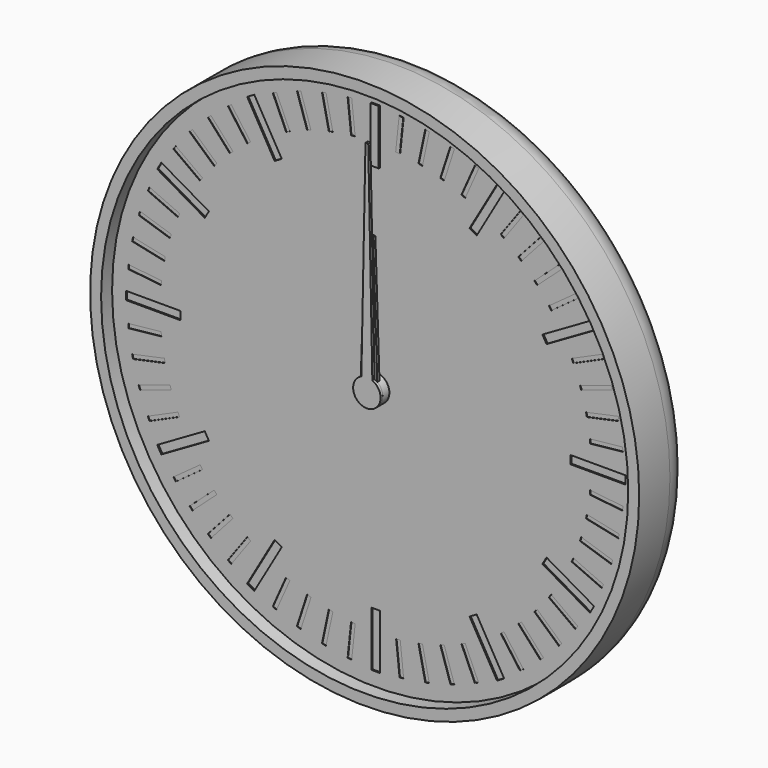
from build123d import *

# Parameters (mm, degrees)
F0_R      = 100
F1_DEPTH  = 24
F2_R      = 10
F3_T      = -4
F4_R      = 5
F4_R_2    = 3
F5_DEPTH  = 2
F6_DEPTH  = 19
F7_DEPTH  = 8
F9_DEPTH  = 4
F11_DEPTH = 4
F12_R     = 5
F12_R_2   = 3
F13_DEPTH = 2
F14_R     = 3
F15_DEPTH = 4
F17_DEPTH = 4
F18_R     = 3
F19_DEPTH = 2
F20_R     = 98
F20_R_2   = 5
F21_DEPTH = 1
F23_R     = 5
F23_R_2   = 3
F24_DEPTH = 2
F25_W     = 3
F25_H     = 20
F25_W_2   = 20
F25_H_2   = 3
F26_DEPTH = 0.5
F27_W     = 1.5
F27_H     = 12
F27_W_2   = 12
F27_H_2   = 1.5
F28_DEPTH = 0.2
F29_DEPTH = 1
F30_DEPTH = 0.4
F31_R     = 5
F31_R_2   = 3
F32_DEPTH = 5
F33_R     = 3
F34_DEPTH = 1
F36_DEPTH = 1


with BuildPart() as f1:
    # F0 (on Front) → F1 (new body)
    with BuildSketch(Plane.XZ):
        Circle(F0_R)
    extrude(amount=F1_DEPTH)

    # F2
    f2_edges = [f1.edges().sort_by_distance(p)[0] for p in [
        (-100, 0, 0),
    ]]
    fillet(f2_edges, radius=F2_R)

    # F3
    f3_openings = [f1.faces().sort_by_distance(p)[0] for p in [
        (0, -24, 0),
    ]]
    offset(amount=F3_T, openings=f3_openings)

    # F4 (on face) → F5 (join)
    with BuildSketch(Plane.XZ.offset(4)):
        Circle(F4_R)
        Circle(F4_R_2, mode=Mode.SUBTRACT)
        with Locations((40, 0)):
            Circle(F4_R)
        with Locations((40, 0)):
            Circle(F4_R_2, mode=Mode.SUBTRACT)
    extrude(amount=F5_DEPTH)


with BuildPart() as f6:
    # F6 (new): a face of the model
    f6_faces = [f1.part.faces().sort_by_distance(p)[0] for p in [
        (0, -4, 0),
    ]]
    extrude(f6_faces, amount=F6_DEPTH)

    # F8 (on face) → F9 (join)
    with BuildSketch(Plane.XZ.offset(6)):
        with BuildLine():
            ThreePointArc((9.2729637667, -1.3794085621), (9.3494561423, -0.6915886375), (9.375, 0))
            ThreePointArc((9.375, 0), (9.3494561423, 0.6915886375), (9.2729637667, 1.3794085621))
            ThreePointArc((9.2729637667, 1.3794085621), (8.9161548403, 2.8970343223), (8.3127812852, 4.3345463782))
            ThreePointArc((8.3127812852, 4.3345463782), (7.5845343223, 5.5104867402), (6.6911892658, 6.566476316))
            ThreePointArc((6.6911892658, 6.566476316), (5.5104867402, 7.5845343223), (4.1773988938, 8.3928519278))
            ThreePointArc((4.1773988938, 8.3928519278), (2.8970343223, 8.9161548403), (1.5536078905, 9.2453733036))
            ThreePointArc((1.5536078905, 9.2453733036), (0, 9.375), (-1.5536078905, 9.2453733036))
            ThreePointArc((-1.5536078905, 9.2453733036), (-2.8970343223, 8.9161548403), (-4.1773988938, 8.3928519278))
            ThreePointArc((-4.1773988938, 8.3928519278), (-5.5104867402, 7.5845343223), (-6.6911892658, 6.566476316))
            ThreePointArc((-6.6911892658, 6.566476316), (-7.5845343223, 5.5104867402), (-8.3127812852, 4.3345463782))
            ThreePointArc((-8.3127812852, 4.3345463782), (-8.9161548403, 2.8970343223), (-9.2729637667, 1.3794085621))
            ThreePointArc((-9.2729637667, 1.3794085621), (-9.375, 0), (-9.2729637667, -1.3794085621))
            ThreePointArc((-9.2729637667, -1.3794085621), (-8.9161548403, -2.8970343223), (-8.3127812852, -4.3345463782))
            ThreePointArc((-8.3127812852, -4.3345463782), (-7.5845343223, -5.5104867402), (-6.6911892658, -6.566476316))
            ThreePointArc((-6.6911892658, -6.566476316), (-5.5104867402, -7.5845343223), (-4.1773988938, -8.3928519278))
            ThreePointArc((-4.1773988938, -8.3928519278), (-2.8970343223, -8.9161548403), (-1.5536078905, -9.2453733036))
            ThreePointArc((-1.5536078905, -9.2453733036), (0, -9.375), (1.5536078905, -9.2453733036))
            ThreePointArc((1.5536078905, -9.2453733036), (2.8970343223, -8.9161548403), (4.1773988938, -8.3928519278))
            ThreePointArc((4.1773988938, -8.3928519278), (5.5104867402, -7.5845343223), (6.6911892658, -6.566476316))
            ThreePointArc((6.6911892658, -6.566476316), (7.5845343223, -5.5104867402), (8.3127812852, -4.3345463782))
            ThreePointArc((8.3127812852, -4.3345463782), (8.9161548403, -2.8970343223), (9.2729637667, -1.3794085621))
        make_face()
        with BuildLine():
            ThreePointArc((8.3127812852, 4.3345463782), (8.9161548403, 2.8970343223), (9.2729637667, 1.3794085621))
            Line((9.2729637667, 1.3794085621), (11.1823199426, 2.3946312492))
            Line((11.1823199426, 2.3946312492), (10.8182678729, 3.515068311))
            Line((10.8182678729, 3.515068311), (10.4542158031, 4.6355053728))
            Line((10.4542158031, 4.6355053728), (8.3127812852, 4.3345463782))
        make_face()
        with BuildLine():
            Line((11.1823199426, -2.3946312492), (9.2729637667, -1.3794085621))
            ThreePointArc((9.2729637667, -1.3794085621), (8.9161548403, -2.8970343223), (8.3127812852, -4.3345463782))
            Line((8.3127812852, -4.3345463782), (10.4542158031, -4.6355053728))
            Line((10.4542158031, -4.6355053728), (10.8182678729, -3.515068311))
            Line((10.8182678729, -3.515068311), (11.1823199426, -2.3946312492))
        make_face()
        with BuildLine():
            ThreePointArc((4.1773988938, 8.3928519278), (5.5104867402, 7.5845343223), (6.6911892658, 6.566476316))
            Line((6.6911892658, 6.566476316), (7.6391579371, 8.5101001246))
            Line((7.6391579371, 8.5101001246), (6.6860572448, 9.202568311))
            Line((6.6860572448, 9.202568311), (5.7329565525, 9.8950364974))
            Line((5.7329565525, 9.8950364974), (4.1773988938, 8.3928519278))
        make_face()
        with BuildLine():
            Line((7.6391579371, -8.5101001246), (6.6911892658, -6.566476316))
            ThreePointArc((6.6911892658, -6.566476316), (5.5104867402, -7.5845343223), (4.1773988938, -8.3928519278))
            Line((4.1773988938, -8.3928519278), (5.7329565525, -9.8950364974))
            Line((5.7329565525, -9.8950364974), (6.6860572448, -9.202568311))
            Line((6.6860572448, -9.202568311), (7.6391579371, -8.5101001246))
        make_face()
        with BuildLine():
            ThreePointArc((-1.5536078905, 9.2453733036), (0, 9.375), (1.5536078905, 9.2453733036))
            Line((1.5536078905, 9.2453733036), (1.1780972451, 11.375))
            Line((1.1780972451, 11.375), (0, 11.375))
            Line((0, 11.375), (-1.1780972451, 11.375))
            Line((-1.1780972451, 11.375), (-1.5536078905, 9.2453733036))
        make_face()
        with BuildLine():
            Line((1.1780972451, -11.375), (1.5536078905, -9.2453733036))
            ThreePointArc((1.5536078905, -9.2453733036), (0, -9.375), (-1.5536078905, -9.2453733036))
            Line((-1.5536078905, -9.2453733036), (-1.1780972451, -11.375))
            Line((-1.1780972451, -11.375), (0, -11.375))
            Line((0, -11.375), (1.1780972451, -11.375))
        make_face()
        with BuildLine():
            ThreePointArc((-6.6911892658, 6.566476316), (-5.5104867402, 7.5845343223), (-4.1773988938, 8.3928519278))
            Line((-4.1773988938, 8.3928519278), (-5.7329565525, 9.8950364974))
            Line((-5.7329565525, 9.8950364974), (-6.6860572448, 9.202568311))
            Line((-6.6860572448, 9.202568311), (-7.6391579371, 8.5101001246))
            Line((-7.6391579371, 8.5101001246), (-6.6911892658, 6.566476316))
        make_face()
        with BuildLine():
            Line((-5.7329565525, -9.8950364974), (-4.1773988938, -8.3928519278))
            ThreePointArc((-4.1773988938, -8.3928519278), (-5.5104867402, -7.5845343223), (-6.6911892658, -6.566476316))
            Line((-6.6911892658, -6.566476316), (-7.6391579371, -8.5101001246))
            Line((-7.6391579371, -8.5101001246), (-6.6860572448, -9.202568311))
            Line((-6.6860572448, -9.202568311), (-5.7329565525, -9.8950364974))
        make_face()
        with BuildLine():
            ThreePointArc((-9.2729637667, 1.3794085621), (-8.9161548403, 2.8970343223), (-8.3127812852, 4.3345463782))
            Line((-8.3127812852, 4.3345463782), (-10.4542158031, 4.6355053728))
            Line((-10.4542158031, 4.6355053728), (-10.8182678729, 3.515068311))
            Line((-10.8182678729, 3.515068311), (-11.1823199426, 2.3946312492))
            Line((-11.1823199426, 2.3946312492), (-9.2729637667, 1.3794085621))
        make_face()
        with BuildLine():
            Line((-10.4542158031, -4.6355053728), (-8.3127812852, -4.3345463782))
            ThreePointArc((-8.3127812852, -4.3345463782), (-8.9161548403, -2.8970343223), (-9.2729637667, -1.3794085621))
            Line((-9.2729637667, -1.3794085621), (-11.1823199426, -2.3946312492))
            Line((-11.1823199426, -2.3946312492), (-10.8182678729, -3.515068311))
            Line((-10.8182678729, -3.515068311), (-10.4542158031, -4.6355053728))
        make_face()
    extrude(amount=F9_DEPTH)

    # F35 (on face) → F36 (join)
    with BuildSketch(Plane.XZ.offset(23)):
        with BuildLine():
            ThreePointArc((-2, 4.582575695), (-2.7386127875, -4.1833001327), (5, 0))
            ThreePointArc((5, 0), (4.1833001327, 2.7386127875), (2, 4.582575695))
            ThreePointArc((2, 4.582575695), (0, 5), (-2, 4.582575695))
        make_face()
        with BuildLine():
            ThreePointArc((-2, 4.582575695), (0, 5), (2, 4.582575695))
            Line((2, 4.582575695), (0.5, 80))
            Line((0.5, 80), (0, 80))
            Line((0, 80), (-0.5, 80))
            Line((-0.5, 80), (-2, 4.582575695))
        make_face()
    extrude(amount=-F36_DEPTH)


with BuildPart() as f7:
    # F7 (new): a face of the model
    f7_faces = [f1.part.faces().sort_by_distance(p)[0] for p in [
        (40, -4, 0),
    ]]
    extrude(f7_faces, amount=F7_DEPTH)

    # F10 (on face) → F11 (join)
    with BuildSketch(Plane.XZ.offset(6)):
        with BuildLine():
            ThreePointArc((68.0829066802, -1.5381733945), (68.1144747006, -0.7693746225), (68.125, 0))
            ThreePointArc((68.125, 0), (68.1144747006, 0.7693746225), (68.0829066802, 1.5381733945))
            ThreePointArc((68.0829066802, 1.5381733945), (67.9709283072, 2.9398630294), (67.7890320221, 4.3342039956))
            ThreePointArc((67.7890320221, 4.3342039956), (67.5104012706, 5.8475163042), (67.1494235596, 7.3433252263))
            ThreePointArc((67.1494235596, 7.3433252263), (66.7484645208, 8.6911029668), (66.280643318, 10.0171558733))
            ThreePointArc((66.280643318, 10.0171558733), (65.6934659962, 11.4394680865), (65.0293803521, 12.8275385085))
            ThreePointArc((65.0293803521, 12.8275385085), (64.3569644814, 14.0625), (63.6236643925, 15.2623099717))
            ThreePointArc((63.6236643925, 15.2623099717), (62.7536029668, 16.5314602207), (61.815433119, 17.7511268046))
            ThreePointArc((61.815433119, 17.7511268046), (60.9009482166, 18.8192983038), (59.934217974, 19.8404278876))
            ThreePointArc((59.934217974, 19.8404278876), (58.8192983038, 20.9009482166), (57.6480467764, 21.8989056799))
            ThreePointArc((57.6480467764, 21.8989056799), (56.5314602207, 22.7536029668), (55.3735505752, 23.5514238999))
            ThreePointArc((55.3735505752, 23.5514238999), (54.0625, 24.3569644814), (52.709356105, 25.0895972944))
            ThreePointArc((52.709356105, 25.0895972944), (51.4394680865, 25.6934659962), (50.1409852457, 26.2331096755))
            ThreePointArc((50.1409852457, 26.2331096755), (48.6911029668, 26.7484645208), (47.2152055856, 27.1837531139))
            ThreePointArc((47.2152055856, 27.1837531139), (45.8475163042, 27.5104012706), (44.4652101991, 27.7682826779))
            ThreePointArc((44.4652101991, 27.7682826779), (42.9398630294, 27.9709283072), (41.4057159597, 28.0898484802))
            ThreePointArc((41.4057159597, 28.0898484802), (40, 28.125), (38.5942840403, 28.0898484802))
            ThreePointArc((38.5942840403, 28.0898484802), (37.0601369706, 27.9709283072), (35.5347898009, 27.7682826779))
            ThreePointArc((35.5347898009, 27.7682826779), (34.1524836958, 27.5104012706), (32.7847944144, 27.1837531139))
            ThreePointArc((32.7847944144, 27.1837531139), (31.3088970332, 26.7484645208), (29.8590147543, 26.2331096755))
            ThreePointArc((29.8590147543, 26.2331096755), (28.5605319135, 25.6934659962), (27.290643895, 25.0895972944))
            ThreePointArc((27.290643895, 25.0895972944), (25.9375, 24.3569644814), (24.6264494248, 23.5514238999))
            ThreePointArc((24.6264494248, 23.5514238999), (23.4685397793, 22.7536029668), (22.3519532236, 21.8989056799))
            ThreePointArc((22.3519532236, 21.8989056799), (21.1807016962, 20.9009482166), (20.065782026, 19.8404278876))
            ThreePointArc((20.065782026, 19.8404278876), (19.0990517834, 18.8192983038), (18.184566881, 17.7511268046))
            ThreePointArc((18.184566881, 17.7511268046), (17.2463970332, 16.5314602207), (16.3763356075, 15.2623099717))
            ThreePointArc((16.3763356075, 15.2623099717), (15.6430355186, 14.0625), (14.9706196479, 12.8275385085))
            ThreePointArc((14.9706196479, 12.8275385085), (14.3065340038, 11.4394680865), (13.719356682, 10.0171558733))
            ThreePointArc((13.719356682, 10.0171558733), (13.2515354792, 8.6911029668), (12.8505764404, 7.3433252263))
            ThreePointArc((12.8505764404, 7.3433252263), (12.4895987294, 5.8475163042), (12.2109679779, 4.3342039956))
            ThreePointArc((12.2109679779, 4.3342039956), (12.0290716928, 2.9398630294), (11.9170933198, 1.5381733945))
            ThreePointArc((11.9170933198, 1.5381733945), (11.875, 0), (11.9170933198, -1.5381733945))
            ThreePointArc((11.9170933198, -1.5381733945), (12.0290716928, -2.9398630294), (12.2109679779, -4.3342039956))
            ThreePointArc((12.2109679779, -4.3342039956), (12.4895987294, -5.8475163042), (12.8505764404, -7.3433252263))
            ThreePointArc((12.8505764404, -7.3433252263), (13.2515354792, -8.6911029668), (13.719356682, -10.0171558733))
            ThreePointArc((13.719356682, -10.0171558733), (14.3065340038, -11.4394680865), (14.9706196479, -12.8275385085))
            ThreePointArc((14.9706196479, -12.8275385085), (15.6430355186, -14.0625), (16.3763356075, -15.2623099717))
            ThreePointArc((16.3763356075, -15.2623099717), (17.2463970332, -16.5314602207), (18.184566881, -17.7511268046))
            ThreePointArc((18.184566881, -17.7511268046), (19.0990517834, -18.8192983038), (20.065782026, -19.8404278876))
            ThreePointArc((20.065782026, -19.8404278876), (21.1807016962, -20.9009482166), (22.3519532236, -21.8989056799))
            ThreePointArc((22.3519532236, -21.8989056799), (23.4685397793, -22.7536029668), (24.6264494248, -23.5514238999))
            ThreePointArc((24.6264494248, -23.5514238999), (25.9375, -24.3569644814), (27.290643895, -25.0895972944))
            ThreePointArc((27.290643895, -25.0895972944), (28.5605319135, -25.6934659962), (29.8590147543, -26.2331096755))
            ThreePointArc((29.8590147543, -26.2331096755), (31.3088970332, -26.7484645208), (32.7847944144, -27.1837531139))
            ThreePointArc((32.7847944144, -27.1837531139), (34.1524836958, -27.5104012706), (35.5347898009, -27.7682826779))
            ThreePointArc((35.5347898009, -27.7682826779), (37.0601369706, -27.9709283072), (38.5942840403, -28.0898484802))
            ThreePointArc((38.5942840403, -28.0898484802), (40, -28.125), (41.4057159597, -28.0898484802))
            ThreePointArc((41.4057159597, -28.0898484802), (42.9398630294, -27.9709283072), (44.4652101991, -27.7682826779))
            ThreePointArc((44.4652101991, -27.7682826779), (45.8475163042, -27.5104012706), (47.2152055856, -27.1837531139))
            ThreePointArc((47.2152055856, -27.1837531139), (48.6911029668, -26.7484645208), (50.1409852457, -26.2331096755))
            ThreePointArc((50.1409852457, -26.2331096755), (51.4394680865, -25.6934659962), (52.709356105, -25.0895972944))
            ThreePointArc((52.709356105, -25.0895972944), (54.0625, -24.3569644814), (55.3735505752, -23.5514238999))
            ThreePointArc((55.3735505752, -23.5514238999), (56.5314602207, -22.7536029668), (57.6480467764, -21.8989056799))
            ThreePointArc((57.6480467764, -21.8989056799), (58.8192983038, -20.9009482166), (59.934217974, -19.8404278876))
            ThreePointArc((59.934217974, -19.8404278876), (60.9009482166, -18.8192983038), (61.815433119, -17.7511268046))
            ThreePointArc((61.815433119, -17.7511268046), (62.7536029668, -16.5314602207), (63.6236643925, -15.2623099717))
            ThreePointArc((63.6236643925, -15.2623099717), (64.3569644814, -14.0625), (65.0293803521, -12.8275385085))
            ThreePointArc((65.0293803521, -12.8275385085), (65.6934659962, -11.4394680865), (66.280643318, -10.0171558733))
            ThreePointArc((66.280643318, -10.0171558733), (66.7484645208, -8.6911029668), (67.1494235596, -7.3433252263))
            ThreePointArc((67.1494235596, -7.3433252263), (67.5104012706, -5.8475163042), (67.7890320221, -4.3342039956))
            ThreePointArc((67.7890320221, -4.3342039956), (67.9709283072, -2.9398630294), (68.0829066802, -1.5381733945))
        make_face()
        with BuildLine():
            ThreePointArc((68.0829066802, 1.5381733945), (68.1144747006, 0.7693746225), (68.125, 0))
            ThreePointArc((68.125, 0), (68.1144747006, -0.7693746225), (68.0829066802, -1.5381733945))
            Line((68.0829066802, -1.5381733945), (70.125, -1.1780972451))
            Line((70.125, -1.1780972451), (70.125, 0))
            Line((70.125, 0), (70.125, 1.1780972451))
            Line((70.125, 1.1780972451), (68.0829066802, 1.5381733945))
        make_face()
        with BuildLine():
            ThreePointArc((67.1494235596, 7.3433252263), (67.5104012706, 5.8475163042), (67.7890320221, 4.3342039956))
            Line((67.7890320221, 4.3342039956), (69.7116366623, 5.1109866922))
            Line((69.7116366623, 5.1109866922), (69.4666964721, 6.2633396859))
            Line((69.4666964721, 6.2633396859), (69.2217562819, 7.4156926796))
            Line((69.2217562819, 7.4156926796), (67.1494235596, 7.3433252263))
        make_face()
        with BuildLine():
            Line((69.7116366623, -5.1109866922), (67.7890320221, -4.3342039956))
            ThreePointArc((67.7890320221, -4.3342039956), (67.5104012706, -5.8475163042), (67.1494235596, -7.3433252263))
            Line((67.1494235596, -7.3433252263), (69.2217562819, -7.4156926796))
            Line((69.2217562819, -7.4156926796), (69.4666964721, -6.2633396859))
            Line((69.4666964721, -6.2633396859), (69.7116366623, -5.1109866922))
        make_face()
        with BuildLine():
            ThreePointArc((65.0293803521, 12.8275385085), (65.6934659962, 11.4394680865), (66.280643318, 10.0171558733))
            Line((66.280643318, 10.0171558733), (67.9997322302, 11.1766959857))
            Line((67.9997322302, 11.1766959857), (67.5205569115, 12.2529413727))
            Line((67.5205569115, 12.2529413727), (67.0413815928, 13.3291867596))
            Line((67.0413815928, 13.3291867596), (65.0293803521, 12.8275385085))
        make_face()
        with BuildLine():
            Line((67.9997322302, -11.1766959857), (66.280643318, -10.0171558733))
            ThreePointArc((66.280643318, -10.0171558733), (65.6934659962, -11.4394680865), (65.0293803521, -12.8275385085))
            Line((65.0293803521, -12.8275385085), (67.0413815928, -13.3291867596))
            Line((67.0413815928, -13.3291867596), (67.5205569115, -12.2529413727))
            Line((67.5205569115, -12.2529413727), (67.9997322302, -11.1766959857))
        make_face()
        with BuildLine():
            ThreePointArc((61.815433119, 17.7511268046), (62.7536029668, 16.5314602207), (63.6236643925, 15.2623099717))
            Line((63.6236643925, 15.2623099717), (65.064105142, 16.753930033))
            Line((65.064105142, 16.753930033), (64.3716369555, 17.7070307253))
            Line((64.3716369555, 17.7070307253), (63.6791687691, 18.6601314176))
            Line((63.6791687691, 18.6601314176), (61.815433119, 17.7511268046))
        make_face()
        with BuildLine():
            Line((65.064105142, -16.753930033), (63.6236643925, -15.2623099717))
            ThreePointArc((63.6236643925, -15.2623099717), (62.7536029668, -16.5314602207), (61.815433119, -17.7511268046))
            Line((61.815433119, -17.7511268046), (63.6791687691, -18.6601314176))
            Line((63.6791687691, -18.6601314176), (64.3716369555, -17.7070307253))
            Line((64.3716369555, -17.7070307253), (65.064105142, -16.753930033))
        make_face()
        with BuildLine():
            ThreePointArc((57.6480467764, 21.8989056799), (58.8192983038, 20.9009482166), (59.934217974, 19.8404278876))
            Line((59.934217974, 19.8404278876), (61.0330563882, 21.5989369435))
            Line((61.0330563882, 21.5989369435), (60.1575595166, 22.3872378675))
            Line((60.1575595166, 22.3872378675), (59.282062645, 23.1755387915))
            Line((59.282062645, 23.1755387915), (57.6480467764, 21.8989056799))
        make_face()
        with BuildLine():
            Line((61.0330563882, -21.5989369435), (59.934217974, -19.8404278876))
            ThreePointArc((59.934217974, -19.8404278876), (58.8192983038, -20.9009482166), (57.6480467764, -21.8989056799))
            Line((57.6480467764, -21.8989056799), (59.282062645, -23.1755387915))
            Line((59.282062645, -23.1755387915), (60.1575595166, -22.3872378675))
            Line((60.1575595166, -22.3872378675), (61.0330563882, -21.5989369435))
        make_face()
        with BuildLine():
            ThreePointArc((52.709356105, 25.0895972944), (54.0625, 24.3569644814), (55.3735505752, 23.5514238999))
            Line((55.3735505752, 23.5514238999), (56.0827621424, 25.4999666665))
            Line((56.0827621424, 25.4999666665), (55.0625, 26.089015289))
            Line((55.0625, 26.089015289), (54.0422378576, 26.6780639116))
            Line((54.0422378576, 26.6780639116), (52.709356105, 25.0895972944))
        make_face()
        with BuildLine():
            Line((56.0827621424, -25.4999666665), (55.3735505752, -23.5514238999))
            ThreePointArc((55.3735505752, -23.5514238999), (54.0625, -24.3569644814), (52.709356105, -25.0895972944))
            Line((52.709356105, -25.0895972944), (54.0422378576, -26.6780639116))
            Line((54.0422378576, -26.6780639116), (55.0625, -26.089015289))
            Line((55.0625, -26.089015289), (56.0827621424, -25.4999666665))
        make_face()
        with BuildLine():
            ThreePointArc((47.2152055856, 27.1837531139), (48.6911029668, 26.7484645208), (50.1409852457, 26.2331096755))
            Line((50.1409852457, 26.2331096755), (50.4295740173, 28.2865254836))
            Line((50.4295740173, 28.2865254836), (49.3091369555, 28.6505775534))
            Line((49.3091369555, 28.6505775534), (48.1886998938, 29.0146296232))
            Line((48.1886998938, 29.0146296232), (47.2152055856, 27.1837531139))
        make_face()
        with BuildLine():
            Line((50.4295740173, -28.2865254836), (50.1409852457, -26.2331096755))
            ThreePointArc((50.1409852457, -26.2331096755), (48.6911029668, -26.7484645208), (47.2152055856, -27.1837531139))
            Line((47.2152055856, -27.1837531139), (48.1886998938, -29.0146296232))
            Line((48.1886998938, -29.0146296232), (49.3091369555, -28.6505775534))
            Line((49.3091369555, -28.6505775534), (50.4295740173, -28.2865254836))
        make_face()
        with BuildLine():
            ThreePointArc((41.4057159597, 28.0898484802), (42.9398630294, 27.9709283072), (44.4652101991, 27.7682826779))
            Line((44.4652101991, 27.7682826779), (44.3205634611, 29.8368274034))
            Line((44.3205634611, 29.8368274034), (43.1489199559, 29.959972098))
            Line((43.1489199559, 29.959972098), (41.9772764508, 30.0831167926))
            Line((41.9772764508, 30.0831167926), (41.4057159597, 28.0898484802))
        make_face()
        with BuildLine():
            Line((44.3205634611, -29.8368274034), (44.4652101991, -27.7682826779))
            ThreePointArc((44.4652101991, -27.7682826779), (42.9398630294, -27.9709283072), (41.4057159597, -28.0898484802))
            Line((41.4057159597, -28.0898484802), (41.9772764508, -30.0831167926))
            Line((41.9772764508, -30.0831167926), (43.1489199559, -29.959972098))
            Line((43.1489199559, -29.959972098), (44.3205634611, -29.8368274034))
        make_face()
        with BuildLine():
            ThreePointArc((35.5347898009, 27.7682826779), (37.0601369706, 27.9709283072), (38.5942840403, 28.0898484802))
            Line((38.5942840403, 28.0898484802), (38.0227235492, 30.0831167926))
            Line((38.0227235492, 30.0831167926), (36.8510800441, 29.959972098))
            Line((36.8510800441, 29.959972098), (35.6794365389, 29.8368274034))
            Line((35.6794365389, 29.8368274034), (35.5347898009, 27.7682826779))
        make_face()
        with BuildLine():
            Line((38.0227235492, -30.0831167926), (38.5942840403, -28.0898484802))
            ThreePointArc((38.5942840403, -28.0898484802), (37.0601369706, -27.9709283072), (35.5347898009, -27.7682826779))
            Line((35.5347898009, -27.7682826779), (35.6794365389, -29.8368274034))
            Line((35.6794365389, -29.8368274034), (36.8510800441, -29.959972098))
            Line((36.8510800441, -29.959972098), (38.0227235492, -30.0831167926))
        make_face()
        with BuildLine():
            ThreePointArc((29.8590147543, 26.2331096755), (31.3088970332, 26.7484645208), (32.7847944144, 27.1837531139))
            Line((32.7847944144, 27.1837531139), (31.8113001062, 29.0146296232))
            Line((31.8113001062, 29.0146296232), (30.6908630445, 28.6505775534))
            Line((30.6908630445, 28.6505775534), (29.5704259827, 28.2865254836))
            Line((29.5704259827, 28.2865254836), (29.8590147543, 26.2331096755))
        make_face()
        with BuildLine():
            Line((31.8113001062, -29.0146296232), (32.7847944144, -27.1837531139))
            ThreePointArc((32.7847944144, -27.1837531139), (31.3088970332, -26.7484645208), (29.8590147543, -26.2331096755))
            Line((29.8590147543, -26.2331096755), (29.5704259827, -28.2865254836))
            Line((29.5704259827, -28.2865254836), (30.6908630445, -28.6505775534))
            Line((30.6908630445, -28.6505775534), (31.8113001062, -29.0146296232))
        make_face()
        with BuildLine():
            ThreePointArc((24.6264494248, 23.5514238999), (25.9375, 24.3569644814), (27.290643895, 25.0895972944))
            Line((27.290643895, 25.0895972944), (25.9577621424, 26.6780639116))
            Line((25.9577621424, 26.6780639116), (24.9375, 26.089015289))
            Line((24.9375, 26.089015289), (23.9172378576, 25.4999666665))
            Line((23.9172378576, 25.4999666665), (24.6264494248, 23.5514238999))
        make_face()
        with BuildLine():
            Line((25.9577621424, -26.6780639116), (27.290643895, -25.0895972944))
            ThreePointArc((27.290643895, -25.0895972944), (25.9375, -24.3569644814), (24.6264494248, -23.5514238999))
            Line((24.6264494248, -23.5514238999), (23.9172378576, -25.4999666665))
            Line((23.9172378576, -25.4999666665), (24.9375, -26.089015289))
            Line((24.9375, -26.089015289), (25.9577621424, -26.6780639116))
        make_face()
        with BuildLine():
            ThreePointArc((20.065782026, 19.8404278876), (21.1807016962, 20.9009482166), (22.3519532236, 21.8989056799))
            Line((22.3519532236, 21.8989056799), (20.717937355, 23.1755387915))
            Line((20.717937355, 23.1755387915), (19.8424404834, 22.3872378675))
            Line((19.8424404834, 22.3872378675), (18.9669436118, 21.5989369435))
            Line((18.9669436118, 21.5989369435), (20.065782026, 19.8404278876))
        make_face()
        with BuildLine():
            Line((20.717937355, -23.1755387915), (22.3519532236, -21.8989056799))
            ThreePointArc((22.3519532236, -21.8989056799), (21.1807016962, -20.9009482166), (20.065782026, -19.8404278876))
            Line((20.065782026, -19.8404278876), (18.9669436118, -21.5989369435))
            Line((18.9669436118, -21.5989369435), (19.8424404834, -22.3872378675))
            Line((19.8424404834, -22.3872378675), (20.717937355, -23.1755387915))
        make_face()
        with BuildLine():
            ThreePointArc((16.3763356075, 15.2623099717), (17.2463970332, 16.5314602207), (18.184566881, 17.7511268046))
            Line((18.184566881, 17.7511268046), (16.3208312309, 18.6601314176))
            Line((16.3208312309, 18.6601314176), (15.6283630445, 17.7070307253))
            Line((15.6283630445, 17.7070307253), (14.935894858, 16.753930033))
            Line((14.935894858, 16.753930033), (16.3763356075, 15.2623099717))
        make_face()
        with BuildLine():
            Line((16.3208312309, -18.6601314176), (18.184566881, -17.7511268046))
            ThreePointArc((18.184566881, -17.7511268046), (17.2463970332, -16.5314602207), (16.3763356075, -15.2623099717))
            Line((16.3763356075, -15.2623099717), (14.935894858, -16.753930033))
            Line((14.935894858, -16.753930033), (15.6283630445, -17.7070307253))
            Line((15.6283630445, -17.7070307253), (16.3208312309, -18.6601314176))
        make_face()
        with BuildLine():
            ThreePointArc((13.719356682, 10.0171558733), (14.3065340038, 11.4394680865), (14.9706196479, 12.8275385085))
            Line((14.9706196479, 12.8275385085), (12.9586184072, 13.3291867596))
            Line((12.9586184072, 13.3291867596), (12.4794430885, 12.2529413727))
            Line((12.4794430885, 12.2529413727), (12.0002677698, 11.1766959857))
            Line((12.0002677698, 11.1766959857), (13.719356682, 10.0171558733))
        make_face()
        with BuildLine():
            Line((12.9586184072, -13.3291867596), (14.9706196479, -12.8275385085))
            ThreePointArc((14.9706196479, -12.8275385085), (14.3065340038, -11.4394680865), (13.719356682, -10.0171558733))
            Line((13.719356682, -10.0171558733), (12.0002677698, -11.1766959857))
            Line((12.0002677698, -11.1766959857), (12.4794430885, -12.2529413727))
            Line((12.4794430885, -12.2529413727), (12.9586184072, -13.3291867596))
        make_face()
        with BuildLine():
            ThreePointArc((12.2109679779, 4.3342039956), (12.4895987294, 5.8475163042), (12.8505764404, 7.3433252263))
            Line((12.8505764404, 7.3433252263), (10.7782437181, 7.4156926796))
            Line((10.7782437181, 7.4156926796), (10.5333035279, 6.2633396859))
            Line((10.5333035279, 6.2633396859), (10.2883633377, 5.1109866922))
            Line((10.2883633377, 5.1109866922), (12.2109679779, 4.3342039956))
        make_face()
        with BuildLine():
            Line((10.7782437181, -7.4156926796), (12.8505764404, -7.3433252263))
            ThreePointArc((12.8505764404, -7.3433252263), (12.4895987294, -5.8475163042), (12.2109679779, -4.3342039956))
            Line((12.2109679779, -4.3342039956), (10.2883633377, -5.1109866922))
            Line((10.2883633377, -5.1109866922), (10.5333035279, -6.2633396859))
            Line((10.5333035279, -6.2633396859), (10.7782437181, -7.4156926796))
        make_face()
        with BuildLine():
            ThreePointArc((11.9170933198, -1.5381733945), (11.875, 0), (11.9170933198, 1.5381733945))
            Line((11.9170933198, 1.5381733945), (9.875, 1.1780972451))
            Line((9.875, 1.1780972451), (9.875, 0))
            Line((9.875, 0), (9.875, -1.1780972451))
            Line((9.875, -1.1780972451), (11.9170933198, -1.5381733945))
        make_face()
    extrude(amount=F11_DEPTH)

    # F16 (on face) → F17 (join)
    with BuildSketch(Plane.XZ.offset(12)):
        with BuildLine():
            ThreePointArc((47.4288750323, -1.0304444454), (47.4821976298, -0.5164480894), (47.5, 0))
            ThreePointArc((47.5, 0), (47.4821976298, 0.5164480894), (47.4288750323, 1.0304444454))
            ThreePointArc((47.4288750323, 1.0304444454), (47.1329238722, 2.3176274578), (46.6157661985, 3.532936117))
            ThreePointArc((46.6157661985, 3.532936117), (46.0676274578, 4.4083893922), (45.4044061018, 5.2002302532))
            ThreePointArc((45.4044061018, 5.2002302532), (44.4083893922, 6.0676274578), (43.2756595386, 6.7468551628))
            ThreePointArc((43.2756595386, 6.7468551628), (42.3176274578, 7.1329238722), (41.3156377295, 7.3837048536))
            ThreePointArc((41.3156377295, 7.3837048536), (40, 7.5), (38.6843622705, 7.3837048536))
            ThreePointArc((38.6843622705, 7.3837048536), (37.6823725422, 7.1329238722), (36.7243404614, 6.7468551628))
            ThreePointArc((36.7243404614, 6.7468551628), (35.5916106078, 6.0676274578), (34.5955938982, 5.2002302532))
            ThreePointArc((34.5955938982, 5.2002302532), (33.9323725422, 4.4083893922), (33.3842338015, 3.532936117))
            ThreePointArc((33.3842338015, 3.532936117), (32.8670761278, 2.3176274578), (32.5711249677, 1.0304444454))
            ThreePointArc((32.5711249677, 1.0304444454), (32.5, 0), (32.5711249677, -1.0304444454))
            ThreePointArc((32.5711249677, -1.0304444454), (32.8670761278, -2.3176274578), (33.3842338015, -3.532936117))
            ThreePointArc((33.3842338015, -3.532936117), (33.9323725422, -4.4083893922), (34.5955938982, -5.2002302532))
            ThreePointArc((34.5955938982, -5.2002302532), (35.5916106078, -6.0676274578), (36.7243404614, -6.7468551628))
            ThreePointArc((36.7243404614, -6.7468551628), (37.6823725422, -7.1329238722), (38.6843622705, -7.3837048536))
            ThreePointArc((38.6843622705, -7.3837048536), (40, -7.5), (41.3156377295, -7.3837048536))
            ThreePointArc((41.3156377295, -7.3837048536), (42.3176274578, -7.1329238722), (43.2756595386, -6.7468551628))
            ThreePointArc((43.2756595386, -6.7468551628), (44.4083893922, -6.0676274578), (45.4044061018, -5.2002302532))
            ThreePointArc((45.4044061018, -5.2002302532), (46.0676274578, -4.4083893922), (46.6157661985, -3.532936117))
            ThreePointArc((46.6157661985, -3.532936117), (47.1329238722, -2.3176274578), (47.4288750323, -1.0304444454))
        make_face()
        with BuildLine():
            ThreePointArc((46.6157661985, 3.532936117), (47.1329238722, 2.3176274578), (47.4288750323, 1.0304444454))
            Line((47.4288750323, 1.0304444454), (49.3262785606, 2.0393117971))
            Line((49.3262785606, 2.0393117971), (48.743795249, 3.832011096))
            Line((48.743795249, 3.832011096), (46.6157661985, 3.532936117))
        make_face()
        with BuildLine():
            Line((49.3262785606, -2.0393117971), (47.4288750323, -1.0304444454))
            ThreePointArc((47.4288750323, -1.0304444454), (47.1329238722, -2.3176274578), (46.6157661985, -3.532936117))
            Line((46.6157661985, -3.532936117), (48.743795249, -3.832011096))
            Line((48.743795249, -3.832011096), (49.3262785606, -2.0393117971))
        make_face()
        with BuildLine():
            ThreePointArc((43.2756595386, 6.7468551628), (44.4083893922, 6.0676274578), (45.4044061018, 5.2002302532))
            Line((45.4044061018, 5.2002302532), (46.3464404506, 7.1316868974))
            Line((46.3464404506, 7.1316868974), (44.8214793429, 8.2396359957))
            Line((44.8214793429, 8.2396359957), (43.2756595386, 6.7468551628))
        make_face()
        with BuildLine():
            Line((46.3464404506, -7.1316868974), (45.4044061018, -5.2002302532))
            ThreePointArc((45.4044061018, -5.2002302532), (44.4083893922, -6.0676274578), (43.2756595386, -6.7468551628))
            Line((43.2756595386, -6.7468551628), (44.8214793429, -8.2396359957))
            Line((44.8214793429, -8.2396359957), (46.3464404506, -7.1316868974))
        make_face()
        with BuildLine():
            ThreePointArc((38.6843622705, 7.3837048536), (40, 7.5), (41.3156377295, 7.3837048536))
            Line((41.3156377295, 7.3837048536), (40.9424777961, 9.5))
            Line((40.9424777961, 9.5), (39.0575222039, 9.5))
            Line((39.0575222039, 9.5), (38.6843622705, 7.3837048536))
        make_face()
        with BuildLine():
            Line((40.9424777961, -9.5), (41.3156377295, -7.3837048536))
            ThreePointArc((41.3156377295, -7.3837048536), (40, -7.5), (38.6843622705, -7.3837048536))
            Line((38.6843622705, -7.3837048536), (39.0575222039, -9.5))
            Line((39.0575222039, -9.5), (40.9424777961, -9.5))
        make_face()
        with BuildLine():
            ThreePointArc((34.5955938982, 5.2002302532), (35.5916106078, 6.0676274578), (36.7243404614, 6.7468551628))
            Line((36.7243404614, 6.7468551628), (35.1785206571, 8.2396359957))
            Line((35.1785206571, 8.2396359957), (33.6535595494, 7.1316868974))
            Line((33.6535595494, 7.1316868974), (34.5955938982, 5.2002302532))
        make_face()
        with BuildLine():
            Line((35.1785206571, -8.2396359957), (36.7243404614, -6.7468551628))
            ThreePointArc((36.7243404614, -6.7468551628), (35.5916106078, -6.0676274578), (34.5955938982, -5.2002302532))
            Line((34.5955938982, -5.2002302532), (33.6535595494, -7.1316868974))
            Line((33.6535595494, -7.1316868974), (35.1785206571, -8.2396359957))
        make_face()
        with BuildLine():
            ThreePointArc((32.5711249677, 1.0304444454), (32.8670761278, 2.3176274578), (33.3842338015, 3.532936117))
            Line((33.3842338015, 3.532936117), (31.256204751, 3.832011096))
            Line((31.256204751, 3.832011096), (30.6737214394, 2.0393117971))
            Line((30.6737214394, 2.0393117971), (32.5711249677, 1.0304444454))
        make_face()
        with BuildLine():
            Line((31.256204751, -3.832011096), (33.3842338015, -3.532936117))
            ThreePointArc((33.3842338015, -3.532936117), (32.8670761278, -2.3176274578), (32.5711249677, -1.0304444454))
            Line((32.5711249677, -1.0304444454), (30.6737214394, -2.0393117971))
            Line((30.6737214394, -2.0393117971), (31.256204751, -3.832011096))
        make_face()
    extrude(amount=F17_DEPTH)

    # F18 (on face) → F19 (join)
    with BuildSketch(Plane.XZ.offset(16)):
        with Locations((40, 0)):
            Circle(F18_R)
    extrude(amount=F19_DEPTH)


with BuildPart() as f13:
    # F12 (on face) → F13 (new body)
    with BuildSketch(Plane.XZ.offset(10)):
        Circle(F12_R)
        Circle(F12_R_2, mode=Mode.SUBTRACT)
    extrude(amount=F13_DEPTH)

    # F14 (on face) → F15 (join)
    with BuildSketch(Plane.XZ.offset(12)):
        with BuildLine():
            ThreePointArc((29.9718156995, -1.3001014101), (29.9929530972, -0.6502034357), (30, 0))
            ThreePointArc((30, 0), (29.9929530972, 0.6502034357), (29.9718156995, 1.3001014101))
            ThreePointArc((29.9718156995, 1.3001014101), (29.907520012, 2.3537728718), (29.8061935814, 3.4045299509))
            ThreePointArc((29.8061935814, 3.4045299509), (29.6306502179, 4.6930339512), (29.3994322443, 5.9727199596))
            ThreePointArc((29.3994322443, 5.9727199596), (29.1710976119, 7.0033609157), (28.9066440563, 8.0253304855))
            ThreePointArc((28.9066440563, 8.0253304855), (28.5316954889, 9.2705098312), (28.1031371961, 10.4982703213))
            ThreePointArc((28.1031371961, 10.4982703213), (27.7163859753, 11.480502971), (27.2953170189, 12.448520749))
            ThreePointArc((27.2953170189, 12.448520749), (26.7301957257, 13.6197149922), (26.1148496411, 14.765318426))
            ThreePointArc((26.1148496411, 14.765318426), (25.5792049306, 15.6749569415), (25.0118886885, 16.5651871174))
            ThreePointArc((25.0118886885, 16.5651871174), (24.2705098312, 17.6335575688), (23.4835278178, 18.6687953878))
            ThreePointArc((23.4835278178, 18.6687953878), (22.812178968, 19.4834414499), (22.1125846489, 20.2739636023))
            ThreePointArc((22.1125846489, 20.2739636023), (21.2132034356, 21.2132034356), (20.2739636023, 22.1125846489))
            ThreePointArc((20.2739636023, 22.1125846489), (19.4834414499, 22.812178968), (18.6687953878, 23.4835278178))
            ThreePointArc((18.6687953878, 23.4835278178), (17.6335575688, 24.2705098312), (16.5651871174, 25.0118886885))
            ThreePointArc((16.5651871174, 25.0118886885), (15.6749569415, 25.5792049306), (14.765318426, 26.1148496411))
            ThreePointArc((14.765318426, 26.1148496411), (13.6197149922, 26.7301957257), (12.448520749, 27.2953170189))
            ThreePointArc((12.448520749, 27.2953170189), (11.480502971, 27.7163859753), (10.4982703213, 28.1031371961))
            ThreePointArc((10.4982703213, 28.1031371961), (9.2705098312, 28.5316954889), (8.0253304855, 28.9066440563))
            ThreePointArc((8.0253304855, 28.9066440563), (7.0033609157, 29.1710976119), (5.9727199596, 29.3994322443))
            ThreePointArc((5.9727199596, 29.3994322443), (4.6930339512, 29.6306502179), (3.4045299509, 29.8061935814))
            ThreePointArc((3.4045299509, 29.8061935814), (2.3537728718, 29.907520012), (1.3001014101, 29.9718156995))
            ThreePointArc((1.3001014101, 29.9718156995), (0, 30), (-1.3001014101, 29.9718156995))
            ThreePointArc((-1.3001014101, 29.9718156995), (-2.3537728718, 29.907520012), (-3.4045299509, 29.8061935814))
            ThreePointArc((-3.4045299509, 29.8061935814), (-4.6930339512, 29.6306502179), (-5.9727199596, 29.3994322443))
            ThreePointArc((-5.9727199596, 29.3994322443), (-7.0033609157, 29.1710976119), (-8.0253304855, 28.9066440563))
            ThreePointArc((-8.0253304855, 28.9066440563), (-9.2705098312, 28.5316954889), (-10.4982703213, 28.1031371961))
            ThreePointArc((-10.4982703213, 28.1031371961), (-11.480502971, 27.7163859753), (-12.448520749, 27.2953170189))
            ThreePointArc((-12.448520749, 27.2953170189), (-13.6197149922, 26.7301957257), (-14.765318426, 26.1148496411))
            ThreePointArc((-14.765318426, 26.1148496411), (-15.6749569415, 25.5792049306), (-16.5651871174, 25.0118886885))
            ThreePointArc((-16.5651871174, 25.0118886885), (-17.6335575688, 24.2705098312), (-18.6687953878, 23.4835278178))
            ThreePointArc((-18.6687953878, 23.4835278178), (-19.4834414499, 22.812178968), (-20.2739636023, 22.1125846489))
            ThreePointArc((-20.2739636023, 22.1125846489), (-21.2132034356, 21.2132034356), (-22.1125846489, 20.2739636023))
            ThreePointArc((-22.1125846489, 20.2739636023), (-22.812178968, 19.4834414499), (-23.4835278178, 18.6687953878))
            ThreePointArc((-23.4835278178, 18.6687953878), (-24.2705098312, 17.6335575688), (-25.0118886885, 16.5651871174))
            ThreePointArc((-25.0118886885, 16.5651871174), (-25.5792049306, 15.6749569415), (-26.1148496411, 14.765318426))
            ThreePointArc((-26.1148496411, 14.765318426), (-26.7301957257, 13.6197149922), (-27.2953170189, 12.448520749))
            ThreePointArc((-27.2953170189, 12.448520749), (-27.7163859753, 11.480502971), (-28.1031371961, 10.4982703213))
            ThreePointArc((-28.1031371961, 10.4982703213), (-28.5316954889, 9.2705098312), (-28.9066440563, 8.0253304855))
            ThreePointArc((-28.9066440563, 8.0253304855), (-29.1710976119, 7.0033609157), (-29.3994322443, 5.9727199596))
            ThreePointArc((-29.3994322443, 5.9727199596), (-29.6306502179, 4.6930339512), (-29.8061935814, 3.4045299509))
            ThreePointArc((-29.8061935814, 3.4045299509), (-29.907520012, 2.3537728718), (-29.9718156995, 1.3001014101))
            ThreePointArc((-29.9718156995, 1.3001014101), (-30, 0), (-29.9718156995, -1.3001014101))
            ThreePointArc((-29.9718156995, -1.3001014101), (-29.907520012, -2.3537728718), (-29.8061935814, -3.4045299509))
            ThreePointArc((-29.8061935814, -3.4045299509), (-29.6306502179, -4.6930339512), (-29.3994322443, -5.9727199596))
            ThreePointArc((-29.3994322443, -5.9727199596), (-29.1710976119, -7.0033609157), (-28.9066440563, -8.0253304855))
            ThreePointArc((-28.9066440563, -8.0253304855), (-28.5316954889, -9.2705098312), (-28.1031371961, -10.4982703213))
            ThreePointArc((-28.1031371961, -10.4982703213), (-27.7163859753, -11.480502971), (-27.2953170189, -12.448520749))
            ThreePointArc((-27.2953170189, -12.448520749), (-26.7301957257, -13.6197149922), (-26.1148496411, -14.765318426))
            ThreePointArc((-26.1148496411, -14.765318426), (-25.5792049306, -15.6749569415), (-25.0118886885, -16.5651871174))
            ThreePointArc((-25.0118886885, -16.5651871174), (-24.2705098312, -17.6335575688), (-23.4835278178, -18.6687953878))
            ThreePointArc((-23.4835278178, -18.6687953878), (-22.812178968, -19.4834414499), (-22.1125846489, -20.2739636023))
            ThreePointArc((-22.1125846489, -20.2739636023), (-21.2132034356, -21.2132034356), (-20.2739636023, -22.1125846489))
            ThreePointArc((-20.2739636023, -22.1125846489), (-19.4834414499, -22.812178968), (-18.6687953878, -23.4835278178))
            ThreePointArc((-18.6687953878, -23.4835278178), (-17.6335575688, -24.2705098312), (-16.5651871174, -25.0118886885))
            ThreePointArc((-16.5651871174, -25.0118886885), (-15.6749569415, -25.5792049306), (-14.765318426, -26.1148496411))
            ThreePointArc((-14.765318426, -26.1148496411), (-13.6197149922, -26.7301957257), (-12.448520749, -27.2953170189))
            ThreePointArc((-12.448520749, -27.2953170189), (-11.480502971, -27.7163859753), (-10.4982703213, -28.1031371961))
            ThreePointArc((-10.4982703213, -28.1031371961), (-9.2705098312, -28.5316954889), (-8.0253304855, -28.9066440563))
            ThreePointArc((-8.0253304855, -28.9066440563), (-7.0033609157, -29.1710976119), (-5.9727199596, -29.3994322443))
            ThreePointArc((-5.9727199596, -29.3994322443), (-4.6930339512, -29.6306502179), (-3.4045299509, -29.8061935814))
            ThreePointArc((-3.4045299509, -29.8061935814), (-2.3537728718, -29.907520012), (-1.3001014101, -29.9718156995))
            ThreePointArc((-1.3001014101, -29.9718156995), (0, -30), (1.3001014101, -29.9718156995))
            ThreePointArc((1.3001014101, -29.9718156995), (2.3537728718, -29.907520012), (3.4045299509, -29.8061935814))
            ThreePointArc((3.4045299509, -29.8061935814), (4.6930339512, -29.6306502179), (5.9727199596, -29.3994322443))
            ThreePointArc((5.9727199596, -29.3994322443), (7.0033609157, -29.1710976119), (8.0253304855, -28.9066440563))
            ThreePointArc((8.0253304855, -28.9066440563), (9.2705098312, -28.5316954889), (10.4982703213, -28.1031371961))
            ThreePointArc((10.4982703213, -28.1031371961), (11.480502971, -27.7163859753), (12.448520749, -27.2953170189))
            ThreePointArc((12.448520749, -27.2953170189), (13.6197149922, -26.7301957257), (14.765318426, -26.1148496411))
            ThreePointArc((14.765318426, -26.1148496411), (15.6749569415, -25.5792049306), (16.5651871174, -25.0118886885))
            ThreePointArc((16.5651871174, -25.0118886885), (17.6335575688, -24.2705098312), (18.6687953878, -23.4835278178))
            ThreePointArc((18.6687953878, -23.4835278178), (19.4834414499, -22.812178968), (20.2739636023, -22.1125846489))
            ThreePointArc((20.2739636023, -22.1125846489), (21.2132034356, -21.2132034356), (22.1125846489, -20.2739636023))
            ThreePointArc((22.1125846489, -20.2739636023), (22.812178968, -19.4834414499), (23.4835278178, -18.6687953878))
            ThreePointArc((23.4835278178, -18.6687953878), (24.2705098312, -17.6335575688), (25.0118886885, -16.5651871174))
            ThreePointArc((25.0118886885, -16.5651871174), (25.5792049306, -15.6749569415), (26.1148496411, -14.765318426))
            ThreePointArc((26.1148496411, -14.765318426), (26.7301957257, -13.6197149922), (27.2953170189, -12.448520749))
            ThreePointArc((27.2953170189, -12.448520749), (27.7163859753, -11.480502971), (28.1031371961, -10.4982703213))
            ThreePointArc((28.1031371961, -10.4982703213), (28.5316954889, -9.2705098312), (28.9066440563, -8.0253304855))
            ThreePointArc((28.9066440563, -8.0253304855), (29.1710976119, -7.0033609157), (29.3994322443, -5.9727199596))
            ThreePointArc((29.3994322443, -5.9727199596), (29.6306502179, -4.6930339512), (29.8061935814, -3.4045299509))
            ThreePointArc((29.8061935814, -3.4045299509), (29.907520012, -2.3537728718), (29.9718156995, -1.3001014101))
        make_face()
        Circle(F14_R, mode=Mode.SUBTRACT)
        with BuildLine():
            ThreePointArc((29.9718156995, 1.3001014101), (29.9929530972, 0.6502034357), (30, 0))
            ThreePointArc((30, 0), (29.9929530972, -0.6502034357), (29.9718156995, -1.3001014101))
            Line((29.9718156995, -1.3001014101), (32, -0.9424777961))
            Line((32, -0.9424777961), (32, 0))
            Line((32, 0), (32, 0.9424777961))
            Line((32, 0.9424777961), (29.9718156995, 1.3001014101))
        make_face()
        with BuildLine():
            ThreePointArc((29.3994322443, 5.9727199596), (29.6306502179, 4.6930339512), (29.8061935814, 3.4045299509))
            Line((29.8061935814, 3.4045299509), (31.7534629089, 4.0750285508))
            Line((31.7534629089, 4.0750285508), (31.606026899, 5.0059028813))
            Line((31.606026899, 5.0059028813), (31.4585908892, 5.9367772117))
            Line((31.4585908892, 5.9367772117), (29.3994322443, 5.9727199596))
        make_face()
        with BuildLine():
            Line((31.7534629089, -4.0750285508), (29.8061935814, -3.4045299509))
            ThreePointArc((29.8061935814, -3.4045299509), (29.6306502179, -4.6930339512), (29.3994322443, -5.9727199596))
            Line((29.3994322443, -5.9727199596), (31.4585908892, -5.9367772117))
            Line((31.4585908892, -5.9367772117), (31.606026899, -5.0059028813))
            Line((31.606026899, -5.0059028813), (31.7534629089, -4.0750285508))
        make_face()
        with BuildLine():
            ThreePointArc((28.1031371961, 10.4982703213), (28.5316954889, 9.2705098312), (28.9066440563, 8.0253304855))
            Line((28.9066440563, 8.0253304855), (30.7250501773, 8.9921941706))
            Line((30.7250501773, 8.9921941706), (30.4338085214, 9.88854382))
            Line((30.4338085214, 9.88854382), (30.1425668656, 10.7848934694))
            Line((30.1425668656, 10.7848934694), (28.1031371961, 10.4982703213))
        make_face()
        with BuildLine():
            Line((30.7250501773, -8.9921941706), (28.9066440563, -8.0253304855))
            ThreePointArc((28.9066440563, -8.0253304855), (28.5316954889, -9.2705098312), (28.1031371961, -10.4982703213))
            Line((28.1031371961, -10.4982703213), (30.1425668656, -10.7848934694))
            Line((30.1425668656, -10.7848934694), (30.4338085214, -9.88854382))
            Line((30.4338085214, -9.88854382), (30.7250501773, -8.9921941706))
        make_face()
        with BuildLine():
            ThreePointArc((26.1148496411, 14.765318426), (26.7301957257, 13.6197149922), (27.2953170189, 12.448520749))
            Line((27.2953170189, 12.448520749), (28.9400847397, 13.6879421265))
            Line((28.9400847397, 13.6879421265), (28.512208774, 14.5276959917))
            Line((28.512208774, 14.5276959917), (28.0843328084, 15.3674498569))
            Line((28.0843328084, 15.3674498569), (26.1148496411, 14.765318426))
        make_face()
        with BuildLine():
            Line((28.9400847397, -13.6879421265), (27.2953170189, -12.448520749))
            ThreePointArc((27.2953170189, -12.448520749), (26.7301957257, -13.6197149922), (26.1148496411, -14.765318426))
            Line((26.1148496411, -14.765318426), (28.0843328084, -15.3674498569))
            Line((28.0843328084, -15.3674498569), (28.512208774, -14.5276959917))
            Line((28.512208774, -14.5276959917), (28.9400847397, -13.6879421265))
        make_face()
        with BuildLine():
            ThreePointArc((23.4835278178, 18.6687953878), (24.2705098312, 17.6335575688), (25.0118886885, 16.5651871174))
            Line((25.0118886885, 16.5651871174), (26.4425183691, 18.0466475195))
            Line((26.4425183691, 18.0466475195), (25.88854382, 18.8091280734))
            Line((25.88854382, 18.8091280734), (25.3345692709, 19.5716086272))
            Line((25.3345692709, 19.5716086272), (23.4835278178, 18.6687953878))
        make_face()
        with BuildLine():
            Line((26.4425183691, -18.0466475195), (25.0118886885, -16.5651871174))
            ThreePointArc((25.0118886885, -16.5651871174), (24.2705098312, -17.6335575688), (23.4835278178, -18.6687953878))
            Line((23.4835278178, -18.6687953878), (25.3345692709, -19.5716086272))
            Line((25.3345692709, -19.5716086272), (25.88854382, -18.8091280734))
            Line((25.88854382, -18.8091280734), (26.4425183691, -18.0466475195))
        make_face()
        with BuildLine():
            ThreePointArc((20.2739636023, 22.1125846489), (21.2132034356, 21.2132034356), (22.1125846489, 20.2739636023))
            Line((22.1125846489, 20.2739636023), (23.2938494387, 21.9609845572))
            Line((23.2938494387, 21.9609845572), (22.627416998, 22.627416998))
            Line((22.627416998, 22.627416998), (21.9609845572, 23.2938494387))
            Line((21.9609845572, 23.2938494387), (20.2739636023, 22.1125846489))
        make_face()
        with BuildLine():
            Line((23.2938494387, -21.9609845572), (22.1125846489, -20.2739636023))
            ThreePointArc((22.1125846489, -20.2739636023), (21.2132034356, -21.2132034356), (20.2739636023, -22.1125846489))
            Line((20.2739636023, -22.1125846489), (21.9609845572, -23.2938494387))
            Line((21.9609845572, -23.2938494387), (22.627416998, -22.627416998))
            Line((22.627416998, -22.627416998), (23.2938494387, -21.9609845572))
        make_face()
        with BuildLine():
            ThreePointArc((16.5651871174, 25.0118886885), (17.6335575688, 24.2705098312), (18.6687953878, 23.4835278178))
            Line((18.6687953878, 23.4835278178), (19.5716086272, 25.3345692709))
            Line((19.5716086272, 25.3345692709), (18.8091280734, 25.88854382))
            Line((18.8091280734, 25.88854382), (18.0466475195, 26.4425183691))
            Line((18.0466475195, 26.4425183691), (16.5651871174, 25.0118886885))
        make_face()
        with BuildLine():
            Line((19.5716086272, -25.3345692709), (18.6687953878, -23.4835278178))
            ThreePointArc((18.6687953878, -23.4835278178), (17.6335575688, -24.2705098312), (16.5651871174, -25.0118886885))
            Line((16.5651871174, -25.0118886885), (18.0466475195, -26.4425183691))
            Line((18.0466475195, -26.4425183691), (18.8091280734, -25.88854382))
            Line((18.8091280734, -25.88854382), (19.5716086272, -25.3345692709))
        make_face()
        with BuildLine():
            ThreePointArc((12.448520749, 27.2953170189), (13.6197149922, 26.7301957257), (14.765318426, 26.1148496411))
            Line((14.765318426, 26.1148496411), (15.3674498569, 28.0843328084))
            Line((15.3674498569, 28.0843328084), (14.5276959917, 28.512208774))
            Line((14.5276959917, 28.512208774), (13.6879421265, 28.9400847397))
            Line((13.6879421265, 28.9400847397), (12.448520749, 27.2953170189))
        make_face()
        with BuildLine():
            Line((15.3674498569, -28.0843328084), (14.765318426, -26.1148496411))
            ThreePointArc((14.765318426, -26.1148496411), (13.6197149922, -26.7301957257), (12.448520749, -27.2953170189))
            Line((12.448520749, -27.2953170189), (13.6879421265, -28.9400847397))
            Line((13.6879421265, -28.9400847397), (14.5276959917, -28.512208774))
            Line((14.5276959917, -28.512208774), (15.3674498569, -28.0843328084))
        make_face()
        with BuildLine():
            ThreePointArc((8.0253304855, 28.9066440563), (9.2705098312, 28.5316954889), (10.4982703213, 28.1031371961))
            Line((10.4982703213, 28.1031371961), (10.7848934694, 30.1425668656))
            Line((10.7848934694, 30.1425668656), (9.88854382, 30.4338085214))
            Line((9.88854382, 30.4338085214), (8.9921941706, 30.7250501773))
            Line((8.9921941706, 30.7250501773), (8.0253304855, 28.9066440563))
        make_face()
        with BuildLine():
            Line((10.7848934694, -30.1425668656), (10.4982703213, -28.1031371961))
            ThreePointArc((10.4982703213, -28.1031371961), (9.2705098312, -28.5316954889), (8.0253304855, -28.9066440563))
            Line((8.0253304855, -28.9066440563), (8.9921941706, -30.7250501773))
            Line((8.9921941706, -30.7250501773), (9.88854382, -30.4338085214))
            Line((9.88854382, -30.4338085214), (10.7848934694, -30.1425668656))
        make_face()
        with BuildLine():
            ThreePointArc((3.4045299509, 29.8061935814), (4.6930339512, 29.6306502179), (5.9727199596, 29.3994322443))
            Line((5.9727199596, 29.3994322443), (5.9367772117, 31.4585908892))
            Line((5.9367772117, 31.4585908892), (5.0059028813, 31.606026899))
            Line((5.0059028813, 31.606026899), (4.0750285508, 31.7534629089))
            Line((4.0750285508, 31.7534629089), (3.4045299509, 29.8061935814))
        make_face()
        with BuildLine():
            Line((5.9367772117, -31.4585908892), (5.9727199596, -29.3994322443))
            ThreePointArc((5.9727199596, -29.3994322443), (4.6930339512, -29.6306502179), (3.4045299509, -29.8061935814))
            Line((3.4045299509, -29.8061935814), (4.0750285508, -31.7534629089))
            Line((4.0750285508, -31.7534629089), (5.0059028813, -31.606026899))
            Line((5.0059028813, -31.606026899), (5.9367772117, -31.4585908892))
        make_face()
        with BuildLine():
            ThreePointArc((-1.3001014101, 29.9718156995), (0, 30), (1.3001014101, 29.9718156995))
            Line((1.3001014101, 29.9718156995), (0.9424777961, 32))
            Line((0.9424777961, 32), (0, 32))
            Line((0, 32), (-0.9424777961, 32))
            Line((-0.9424777961, 32), (-1.3001014101, 29.9718156995))
        make_face()
        with BuildLine():
            Line((0.9424777961, -32), (1.3001014101, -29.9718156995))
            ThreePointArc((1.3001014101, -29.9718156995), (0, -30), (-1.3001014101, -29.9718156995))
            Line((-1.3001014101, -29.9718156995), (-0.9424777961, -32))
            Line((-0.9424777961, -32), (0, -32))
            Line((0, -32), (0.9424777961, -32))
        make_face()
        with BuildLine():
            ThreePointArc((-5.9727199596, 29.3994322443), (-4.6930339512, 29.6306502179), (-3.4045299509, 29.8061935814))
            Line((-3.4045299509, 29.8061935814), (-4.0750285508, 31.7534629089))
            Line((-4.0750285508, 31.7534629089), (-5.0059028813, 31.606026899))
            Line((-5.0059028813, 31.606026899), (-5.9367772117, 31.4585908892))
            Line((-5.9367772117, 31.4585908892), (-5.9727199596, 29.3994322443))
        make_face()
        with BuildLine():
            Line((-4.0750285508, -31.7534629089), (-3.4045299509, -29.8061935814))
            ThreePointArc((-3.4045299509, -29.8061935814), (-4.6930339512, -29.6306502179), (-5.9727199596, -29.3994322443))
            Line((-5.9727199596, -29.3994322443), (-5.9367772117, -31.4585908892))
            Line((-5.9367772117, -31.4585908892), (-5.0059028813, -31.606026899))
            Line((-5.0059028813, -31.606026899), (-4.0750285508, -31.7534629089))
        make_face()
        with BuildLine():
            ThreePointArc((-10.4982703213, 28.1031371961), (-9.2705098312, 28.5316954889), (-8.0253304855, 28.9066440563))
            Line((-8.0253304855, 28.9066440563), (-8.9921941706, 30.7250501773))
            Line((-8.9921941706, 30.7250501773), (-9.88854382, 30.4338085214))
            Line((-9.88854382, 30.4338085214), (-10.7848934694, 30.1425668656))
            Line((-10.7848934694, 30.1425668656), (-10.4982703213, 28.1031371961))
        make_face()
        with BuildLine():
            Line((-8.9921941706, -30.7250501773), (-8.0253304855, -28.9066440563))
            ThreePointArc((-8.0253304855, -28.9066440563), (-9.2705098312, -28.5316954889), (-10.4982703213, -28.1031371961))
            Line((-10.4982703213, -28.1031371961), (-10.7848934694, -30.1425668656))
            Line((-10.7848934694, -30.1425668656), (-9.88854382, -30.4338085214))
            Line((-9.88854382, -30.4338085214), (-8.9921941706, -30.7250501773))
        make_face()
        with BuildLine():
            ThreePointArc((-14.765318426, 26.1148496411), (-13.6197149922, 26.7301957257), (-12.448520749, 27.2953170189))
            Line((-12.448520749, 27.2953170189), (-13.6879421265, 28.9400847397))
            Line((-13.6879421265, 28.9400847397), (-14.5276959917, 28.512208774))
            Line((-14.5276959917, 28.512208774), (-15.3674498569, 28.0843328084))
            Line((-15.3674498569, 28.0843328084), (-14.765318426, 26.1148496411))
        make_face()
        with BuildLine():
            Line((-13.6879421265, -28.9400847397), (-12.448520749, -27.2953170189))
            ThreePointArc((-12.448520749, -27.2953170189), (-13.6197149922, -26.7301957257), (-14.765318426, -26.1148496411))
            Line((-14.765318426, -26.1148496411), (-15.3674498569, -28.0843328084))
            Line((-15.3674498569, -28.0843328084), (-14.5276959917, -28.512208774))
            Line((-14.5276959917, -28.512208774), (-13.6879421265, -28.9400847397))
        make_face()
        with BuildLine():
            ThreePointArc((-18.6687953878, 23.4835278178), (-17.6335575688, 24.2705098312), (-16.5651871174, 25.0118886885))
            Line((-16.5651871174, 25.0118886885), (-18.0466475195, 26.4425183691))
            Line((-18.0466475195, 26.4425183691), (-18.8091280734, 25.88854382))
            Line((-18.8091280734, 25.88854382), (-19.5716086272, 25.3345692709))
            Line((-19.5716086272, 25.3345692709), (-18.6687953878, 23.4835278178))
        make_face()
        with BuildLine():
            Line((-18.0466475195, -26.4425183691), (-16.5651871174, -25.0118886885))
            ThreePointArc((-16.5651871174, -25.0118886885), (-17.6335575688, -24.2705098312), (-18.6687953878, -23.4835278178))
            Line((-18.6687953878, -23.4835278178), (-19.5716086272, -25.3345692709))
            Line((-19.5716086272, -25.3345692709), (-18.8091280734, -25.88854382))
            Line((-18.8091280734, -25.88854382), (-18.0466475195, -26.4425183691))
        make_face()
        with BuildLine():
            ThreePointArc((-22.1125846489, 20.2739636023), (-21.2132034356, 21.2132034356), (-20.2739636023, 22.1125846489))
            Line((-20.2739636023, 22.1125846489), (-21.9609845572, 23.2938494387))
            Line((-21.9609845572, 23.2938494387), (-22.627416998, 22.627416998))
            Line((-22.627416998, 22.627416998), (-23.2938494387, 21.9609845572))
            Line((-23.2938494387, 21.9609845572), (-22.1125846489, 20.2739636023))
        make_face()
        with BuildLine():
            Line((-21.9609845572, -23.2938494387), (-20.2739636023, -22.1125846489))
            ThreePointArc((-20.2739636023, -22.1125846489), (-21.2132034356, -21.2132034356), (-22.1125846489, -20.2739636023))
            Line((-22.1125846489, -20.2739636023), (-23.2938494387, -21.9609845572))
            Line((-23.2938494387, -21.9609845572), (-22.627416998, -22.627416998))
            Line((-22.627416998, -22.627416998), (-21.9609845572, -23.2938494387))
        make_face()
        with BuildLine():
            ThreePointArc((-25.0118886885, 16.5651871174), (-24.2705098312, 17.6335575688), (-23.4835278178, 18.6687953878))
            Line((-23.4835278178, 18.6687953878), (-25.3345692709, 19.5716086272))
            Line((-25.3345692709, 19.5716086272), (-25.88854382, 18.8091280734))
            Line((-25.88854382, 18.8091280734), (-26.4425183691, 18.0466475195))
            Line((-26.4425183691, 18.0466475195), (-25.0118886885, 16.5651871174))
        make_face()
        with BuildLine():
            Line((-25.3345692709, -19.5716086272), (-23.4835278178, -18.6687953878))
            ThreePointArc((-23.4835278178, -18.6687953878), (-24.2705098312, -17.6335575688), (-25.0118886885, -16.5651871174))
            Line((-25.0118886885, -16.5651871174), (-26.4425183691, -18.0466475195))
            Line((-26.4425183691, -18.0466475195), (-25.88854382, -18.8091280734))
            Line((-25.88854382, -18.8091280734), (-25.3345692709, -19.5716086272))
        make_face()
        with BuildLine():
            ThreePointArc((-27.2953170189, 12.448520749), (-26.7301957257, 13.6197149922), (-26.1148496411, 14.765318426))
            Line((-26.1148496411, 14.765318426), (-28.0843328084, 15.3674498569))
            Line((-28.0843328084, 15.3674498569), (-28.512208774, 14.5276959917))
            Line((-28.512208774, 14.5276959917), (-28.9400847397, 13.6879421265))
            Line((-28.9400847397, 13.6879421265), (-27.2953170189, 12.448520749))
        make_face()
        with BuildLine():
            Line((-28.0843328084, -15.3674498569), (-26.1148496411, -14.765318426))
            ThreePointArc((-26.1148496411, -14.765318426), (-26.7301957257, -13.6197149922), (-27.2953170189, -12.448520749))
            Line((-27.2953170189, -12.448520749), (-28.9400847397, -13.6879421265))
            Line((-28.9400847397, -13.6879421265), (-28.512208774, -14.5276959917))
            Line((-28.512208774, -14.5276959917), (-28.0843328084, -15.3674498569))
        make_face()
        with BuildLine():
            ThreePointArc((-28.9066440563, 8.0253304855), (-28.5316954889, 9.2705098312), (-28.1031371961, 10.4982703213))
            Line((-28.1031371961, 10.4982703213), (-30.1425668656, 10.7848934694))
            Line((-30.1425668656, 10.7848934694), (-30.4338085214, 9.88854382))
            Line((-30.4338085214, 9.88854382), (-30.7250501773, 8.9921941706))
            Line((-30.7250501773, 8.9921941706), (-28.9066440563, 8.0253304855))
        make_face()
        with BuildLine():
            Line((-30.1425668656, -10.7848934694), (-28.1031371961, -10.4982703213))
            ThreePointArc((-28.1031371961, -10.4982703213), (-28.5316954889, -9.2705098312), (-28.9066440563, -8.0253304855))
            Line((-28.9066440563, -8.0253304855), (-30.7250501773, -8.9921941706))
            Line((-30.7250501773, -8.9921941706), (-30.4338085214, -9.88854382))
            Line((-30.4338085214, -9.88854382), (-30.1425668656, -10.7848934694))
        make_face()
        with BuildLine():
            ThreePointArc((-29.8061935814, 3.4045299509), (-29.6306502179, 4.6930339512), (-29.3994322443, 5.9727199596))
            Line((-29.3994322443, 5.9727199596), (-31.4585908892, 5.9367772117))
            Line((-31.4585908892, 5.9367772117), (-31.606026899, 5.0059028813))
            Line((-31.606026899, 5.0059028813), (-31.7534629089, 4.0750285508))
            Line((-31.7534629089, 4.0750285508), (-29.8061935814, 3.4045299509))
        make_face()
        with BuildLine():
            Line((-31.4585908892, -5.9367772117), (-29.3994322443, -5.9727199596))
            ThreePointArc((-29.3994322443, -5.9727199596), (-29.6306502179, -4.6930339512), (-29.8061935814, -3.4045299509))
            Line((-29.8061935814, -3.4045299509), (-31.7534629089, -4.0750285508))
            Line((-31.7534629089, -4.0750285508), (-31.606026899, -5.0059028813))
            Line((-31.606026899, -5.0059028813), (-31.4585908892, -5.9367772117))
        make_face()
        with BuildLine():
            ThreePointArc((-29.9718156995, -1.3001014101), (-30, 0), (-29.9718156995, 1.3001014101))
            Line((-29.9718156995, 1.3001014101), (-32, 0.9424777961))
            Line((-32, 0.9424777961), (-32, 0))
            Line((-32, 0), (-32, -0.9424777961))
            Line((-32, -0.9424777961), (-29.9718156995, -1.3001014101))
        make_face()
    extrude(amount=F15_DEPTH)

    # F31 (on face) → F32 (join)
    with BuildSketch(Plane.XZ.offset(16)):
        Circle(F31_R)
        Circle(F31_R_2, mode=Mode.SUBTRACT)
    extrude(amount=F32_DEPTH)

    # F33 (on face) → F34 (join)
    with BuildSketch(Plane.XZ.offset(21)):
        with BuildLine():
            ThreePointArc((-3, 4), (-2.2360679775, -4.472135955), (5, 0))
            ThreePointArc((5, 0), (4.472135955, 2.2360679775), (3, 4))
            ThreePointArc((3, 4), (0, 5), (-3, 4))
        make_face()
        Circle(F33_R, mode=Mode.SUBTRACT)
        with BuildLine():
            ThreePointArc((-3, 4), (0, 5), (3, 4))
            Line((3, 4), (1.5, 50))
            Line((1.5, 50), (0, 50))
            Line((0, 50), (-1.5, 50))
            Line((-1.5, 50), (-3, 4))
        make_face()
    extrude(amount=F34_DEPTH)


with BuildPart() as f21:
    # F20 (on face) → F21 (new body)
    with BuildSketch(Plane.XZ.offset(18)):
        Circle(F20_R)
        Circle(F20_R_2, mode=Mode.SUBTRACT)
    extrude(amount=F21_DEPTH)


with BuildPart() as f1_1:
    add(f1.part)

    # F22: cut F21
    add(f21.part, mode=Mode.SUBTRACT)


with BuildPart() as f21_1:
    add(f21.part)

    # F23 (on face) → F24 (join, through all)
    with BuildSketch(Plane(origin=(0, -18, 0), x_dir=(-1, 0, 0), z_dir=(0, 1, 0))):
        with Locations((-40, 0)):
            Circle(F23_R)
        with Locations((-40, 0)):
            Circle(F23_R_2, mode=Mode.SUBTRACT)
    extrude(amount=F24_DEPTH)

    # F25 (on face) → F26 (cut)
    with BuildSketch(Plane.XZ.offset(19)):
        with Locations((0, 81)):
            Rectangle(F25_W, F25_H)
        Polygon((-46.7990381057, 78.0583117444), (-36.7990381057, 60.7378036687), (-34.2009618943, 62.2378036687), (-44.2009618943, 79.5583117444), align=None)
        Polygon((-79.5583117444, 44.2009618943), (-62.2378036687, 34.2009618943), (-60.7378036687, 36.7990381057), (-78.0583117444, 46.7990381057), align=None)
        with Locations((-81, 0)):
            Rectangle(F25_W_2, F25_H_2)
        Polygon((-79.5583117444, -44.2009618943), (-78.0583117444, -46.7990381057), (-60.7378036687, -36.7990381057), (-62.2378036687, -34.2009618943), align=None)
        Polygon((-46.7990381057, -78.0583117444), (-44.2009618943, -79.5583117444), (-34.2009618943, -62.2378036687), (-36.7990381057, -60.7378036687), align=None)
        with Locations((0, -81)):
            Rectangle(F25_W, F25_H)
        Polygon((44.2009618943, -79.5583117444), (46.7990381057, -78.0583117444), (36.7990381057, -60.7378036687), (34.2009618943, -62.2378036687), align=None)
        Polygon((78.0583117444, -46.7990381057), (79.5583117444, -44.2009618943), (62.2378036687, -34.2009618943), (60.7378036687, -36.7990381057), align=None)
        with Locations((81, 0)):
            Rectangle(F25_W_2, F25_H_2)
        Polygon((79.5583117444, 44.2009618943), (78.0583117444, 46.7990381057), (60.7378036687, 36.7990381057), (62.2378036687, 34.2009618943), align=None)
        Polygon((46.7990381057, 78.0583117444), (44.2009618943, 79.5583117444), (34.2009618943, 62.2378036687), (36.7990381057, 60.7378036687), align=None)
    extrude(amount=-F26_DEPTH, mode=Mode.SUBTRACT)

    # F27 (on face) → F28 (cut)
    with BuildSketch(Plane.XZ.offset(19)):
        with Locations((0, 84.5)):
            Rectangle(F27_W, F27_H)
        Polygon((-8.7139345042, 90.0826278783), (-10.2057173472, 89.9258351834), (-8.951375788, 77.991572439), (-7.459592945, 78.1483651339), align=None)
        Polygon((-18.0823973185, 88.6782916345), (-19.5496187196, 88.3664240983), (-17.0546784297, 76.6286528895), (-15.5874570286, 76.9405204257), align=None)
        Polygon((-27.2527456037, 86.3023774705), (-28.6793303782, 85.8388519789), (-24.9711264457, 74.4261737834), (-23.5445416712, 74.889699275), align=None)
        Polygon((-36.1245071051, 82.980916399), (-37.4948252916, 82.3708114343), (-32.6139855747, 71.4082659426), (-31.2436673882, 72.0183709073), align=None)
        Polygon((-44.6004809472, 78.7502990425), (-45.8995190528, 78.0002990425), (-39.8995190528, 67.6079941971), (-38.6004809472, 68.3579941971), align=None)
        Polygon((-52.5878025867, 73.6568769302), (-53.8013280782, 72.7751990517), (-46.7479050507, 63.0669951192), (-45.5343795592, 63.9486729977), align=None)
        Polygon((-59.9989612564, 67.7564546605), (-61.1136784946, 66.7527587509), (-53.0841112183, 57.8350208452), (-51.9693939801, 58.8387167547), align=None)
        Polygon((-66.7527587509, 61.1136784946), (-67.7564546605, 59.9989612564), (-58.8387167547, 51.9693939801), (-57.8350208452, 53.0841112183), align=None)
        Polygon((-72.7751990517, 53.8013280783), (-73.6568769302, 52.5878025867), (-63.9486729977, 45.5343795592), (-63.0669951192, 46.7479050507), align=None)
        Polygon((-78.0002990425, 45.8995190528), (-78.7502990425, 44.6004809472), (-68.3579941971, 38.6004809472), (-67.6079941971, 39.8995190528), align=None)
        Polygon((-82.3708114343, 37.4948252916), (-82.980916399, 36.1245071051), (-72.0183709073, 31.2436673882), (-71.4082659426, 32.6139855747), align=None)
        Polygon((-85.8388519789, 28.6793303782), (-86.3023774705, 27.2527456037), (-74.889699275, 23.5445416712), (-74.4261737834, 24.9711264457), align=None)
        Polygon((-88.3664240983, 19.5496187196), (-88.6782916345, 18.0823973185), (-76.9405204257, 15.5874570286), (-76.6286528895, 17.0546784297), align=None)
        Polygon((-89.9258351834, 10.2057173472), (-90.0826278783, 8.7139345042), (-78.1483651339, 7.459592945), (-77.991572439, 8.951375788), align=None)
        with Locations((-84.5, 0)):
            Rectangle(F27_W_2, F27_H_2)
        Polygon((-90.0826278783, -8.7139345042), (-89.9258351834, -10.2057173472), (-77.991572439, -8.951375788), (-78.1483651339, -7.459592945), align=None)
        Polygon((-88.6782916345, -18.0823973185), (-88.3664240983, -19.5496187196), (-76.6286528895, -17.0546784297), (-76.9405204257, -15.5874570286), align=None)
        Polygon((-86.3023774705, -27.2527456037), (-85.8388519789, -28.6793303782), (-74.4261737834, -24.9711264457), (-74.889699275, -23.5445416712), align=None)
        Polygon((-82.980916399, -36.1245071051), (-82.3708114343, -37.4948252916), (-71.4082659426, -32.6139855747), (-72.0183709073, -31.2436673882), align=None)
        Polygon((-78.7502990425, -44.6004809472), (-78.0002990425, -45.8995190528), (-67.6079941971, -39.8995190528), (-68.3579941971, -38.6004809472), align=None)
        Polygon((-73.6568769302, -52.5878025867), (-72.7751990517, -53.8013280782), (-63.0669951192, -46.7479050507), (-63.9486729977, -45.5343795592), align=None)
        Polygon((-67.7564546605, -59.9989612564), (-66.7527587509, -61.1136784946), (-57.8350208452, -53.0841112183), (-58.8387167547, -51.9693939801), align=None)
        Polygon((-61.1136784946, -66.7527587509), (-59.9989612564, -67.7564546605), (-51.9693939801, -58.8387167547), (-53.0841112183, -57.8350208452), align=None)
        Polygon((-53.8013280783, -72.7751990517), (-52.5878025867, -73.6568769302), (-45.5343795592, -63.9486729977), (-46.7479050507, -63.0669951192), align=None)
        Polygon((-45.8995190528, -78.0002990425), (-44.6004809472, -78.7502990425), (-38.6004809472, -68.3579941971), (-39.8995190528, -67.6079941971), align=None)
        Polygon((-37.4948252916, -82.3708114343), (-36.1245071051, -82.980916399), (-31.2436673882, -72.0183709073), (-32.6139855747, -71.4082659426), align=None)
        Polygon((-28.6793303782, -85.8388519789), (-27.2527456037, -86.3023774705), (-23.5445416712, -74.889699275), (-24.9711264457, -74.4261737834), align=None)
        Polygon((-19.5496187196, -88.3664240983), (-18.0823973185, -88.6782916345), (-15.5874570286, -76.9405204257), (-17.0546784297, -76.6286528895), align=None)
        Polygon((-10.2057173472, -89.9258351834), (-8.7139345042, -90.0826278783), (-7.459592945, -78.1483651339), (-8.951375788, -77.991572439), align=None)
        with Locations((0, -84.5)):
            Rectangle(F27_W, F27_H)
        Polygon((8.7139345042, -90.0826278783), (10.2057173472, -89.9258351834), (8.951375788, -77.991572439), (7.459592945, -78.1483651339), align=None)
        Polygon((18.0823973185, -88.6782916345), (19.5496187196, -88.3664240983), (17.0546784297, -76.6286528895), (15.5874570286, -76.9405204257), align=None)
        Polygon((27.2527456037, -86.3023774705), (28.6793303782, -85.8388519789), (24.9711264457, -74.4261737834), (23.5445416712, -74.889699275), align=None)
        Polygon((36.1245071051, -82.980916399), (37.4948252916, -82.3708114343), (32.6139855747, -71.4082659426), (31.2436673882, -72.0183709073), align=None)
        Polygon((44.6004809472, -78.7502990425), (45.8995190528, -78.0002990425), (39.8995190528, -67.6079941971), (38.6004809472, -68.3579941971), align=None)
        Polygon((52.5878025867, -73.6568769302), (53.8013280782, -72.7751990517), (46.7479050507, -63.0669951192), (45.5343795592, -63.9486729977), align=None)
        Polygon((59.9989612564, -67.7564546605), (61.1136784946, -66.7527587509), (53.0841112183, -57.8350208452), (51.9693939801, -58.8387167547), align=None)
        Polygon((66.7527587509, -61.1136784946), (67.7564546605, -59.9989612564), (58.8387167547, -51.9693939801), (57.8350208452, -53.0841112183), align=None)
        Polygon((72.7751990517, -53.8013280783), (73.6568769302, -52.5878025867), (63.9486729977, -45.5343795592), (63.0669951192, -46.7479050507), align=None)
        Polygon((78.0002990425, -45.8995190528), (78.7502990425, -44.6004809472), (68.3579941971, -38.6004809472), (67.6079941971, -39.8995190528), align=None)
        Polygon((82.3708114343, -37.4948252916), (82.980916399, -36.1245071051), (72.0183709073, -31.2436673882), (71.4082659426, -32.6139855747), align=None)
        Polygon((85.8388519789, -28.6793303782), (86.3023774705, -27.2527456037), (74.889699275, -23.5445416712), (74.4261737834, -24.9711264457), align=None)
        Polygon((88.3664240983, -19.5496187196), (88.6782916345, -18.0823973185), (76.9405204257, -15.5874570286), (76.6286528895, -17.0546784297), align=None)
        Polygon((89.9258351834, -10.2057173472), (90.0826278783, -8.7139345042), (78.1483651339, -7.459592945), (77.991572439, -8.951375788), align=None)
        with Locations((84.5, 0)):
            Rectangle(F27_W_2, F27_H_2)
        Polygon((90.0826278783, 8.7139345042), (89.9258351834, 10.2057173472), (77.991572439, 8.951375788), (78.1483651339, 7.459592945), align=None)
        Polygon((88.6782916345, 18.0823973185), (88.3664240983, 19.5496187196), (76.6286528895, 17.0546784297), (76.9405204257, 15.5874570286), align=None)
        Polygon((86.3023774705, 27.2527456037), (85.8388519789, 28.6793303782), (74.4261737834, 24.9711264457), (74.889699275, 23.5445416712), align=None)
        Polygon((82.980916399, 36.1245071051), (82.3708114343, 37.4948252916), (71.4082659426, 32.6139855747), (72.0183709073, 31.2436673882), align=None)
        Polygon((78.7502990425, 44.6004809472), (78.0002990425, 45.8995190528), (67.6079941971, 39.8995190528), (68.3579941971, 38.6004809472), align=None)
        Polygon((73.6568769302, 52.5878025867), (72.7751990517, 53.8013280782), (63.0669951192, 46.7479050507), (63.9486729977, 45.5343795592), align=None)
        Polygon((67.7564546605, 59.9989612564), (66.7527587509, 61.1136784946), (57.8350208452, 53.0841112183), (58.8387167547, 51.9693939801), align=None)
        Polygon((61.1136784946, 66.7527587509), (59.9989612564, 67.7564546605), (51.9693939801, 58.8387167547), (53.0841112183, 57.8350208452), align=None)
        Polygon((53.8013280783, 72.7751990517), (52.5878025867, 73.6568769302), (45.5343795592, 63.9486729977), (46.7479050507, 63.0669951192), align=None)
        Polygon((45.8995190528, 78.0002990425), (44.6004809472, 78.7502990425), (38.6004809472, 68.3579941971), (39.8995190528, 67.6079941971), align=None)
        Polygon((37.4948252916, 82.3708114343), (36.1245071051, 82.980916399), (31.2436673882, 72.0183709073), (32.6139855747, 71.4082659426), align=None)
        Polygon((28.6793303782, 85.8388519789), (27.2527456037, 86.3023774705), (23.5445416712, 74.889699275), (24.9711264457, 74.4261737834), align=None)
        Polygon((19.5496187196, 88.3664240983), (18.0823973185, 88.6782916345), (15.5874570286, 76.9405204257), (17.0546784297, 76.6286528895), align=None)
        Polygon((10.2057173472, 89.9258351834), (8.7139345042, 90.0826278783), (7.459592945, 78.1483651339), (8.951375788, 77.991572439), align=None)
    extrude(amount=-F28_DEPTH, mode=Mode.SUBTRACT)


with BuildPart() as f29:
    # F29 (new): a face of the model
    f29_faces = [f21_1.part.faces().sort_by_distance(p)[0] for p in [
        (0, -18.5, 81),
    ]]
    extrude(f29_faces, amount=F29_DEPTH)


with BuildPart() as f30:
    # F30 (new): a face of the model
    f30_faces = [f21_1.part.faces().sort_by_distance(p)[0] for p in [
        (8.8326551461, -18.8, 84.0371001586),
    ]]
    extrude(f30_faces, amount=F30_DEPTH)


solid = Compound([f6.part, f7.part, f13.part, f1_1.part, f21_1.part, f29.part, f30.part])
